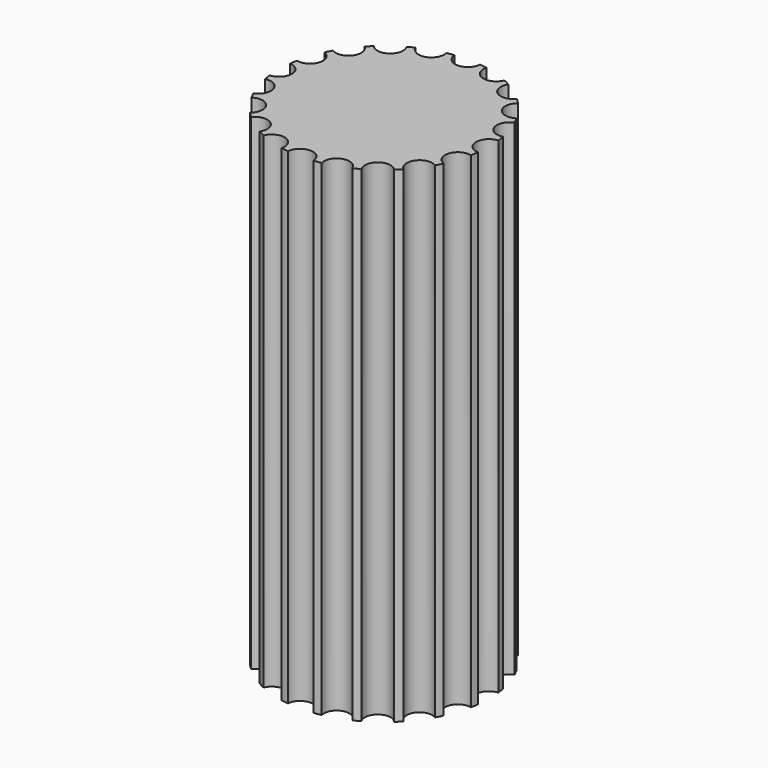
from build123d import *

# Parameters (mm, degrees)
F0_R     = 4.1
F0_R_2   = 3
F1_DEPTH = 19
F3_DEPTH = 25


with BuildPart() as f1:
    # F0 (on Top) → F1 (new body)
    with BuildSketch(Plane.XY):
        Circle(F0_R)
        Circle(F0_R_2, mode=Mode.SUBTRACT)
        Circle(F0_R_2)
    extrude(amount=F1_DEPTH)

    # F2 (on face) → F3 (cut)
    with BuildSketch(Plane.XY.offset(19)):
        with BuildLine():
            ThreePointArc((0.4990696282, 4.0695121951), (0.4997673529, 4.0847490014), (0.5, 4.1))
            ThreePointArc((0.5, 4.1), (-0.0152509986, 4.5997673529), (-0.4990696282, 4.0695121951))
            ThreePointArc((-0.4990696282, 4.0695121951), (0, 4.1), (0.4990696282, 4.0695121951))
        make_face()
        with BuildLine():
            ThreePointArc((0.4990696282, 4.0695121951), (0, 4.1), (-0.4990696282, 4.0695121951))
            ThreePointArc((-0.4990696282, 4.0695121951), (0, 3.6), (0.4990696282, 4.0695121951))
        make_face()
        with BuildLine():
            ThreePointArc((-1.7321918491, 3.7161150948), (-1.2669696769, 3.8993317168), (-0.7829050052, 4.0245570878))
            ThreePointArc((-0.7829050052, 4.0245570878), (-1.4214781741, 4.374859975), (-1.7321918491, 3.7161150948))
        make_face()
        with BuildLine():
            ThreePointArc((-0.7669696769, 3.8993317168), (-0.7709695076, 3.9624493218), (-0.7829050052, 4.0245570878))
            ThreePointArc((-0.7829050052, 4.0245570878), (-1.2669696769, 3.8993317168), (-1.7321918491, 3.7161150948))
            ThreePointArc((-1.7321918491, 3.7161150948), (-1.1737256049, 3.4081031111), (-0.7669696769, 3.8993317168))
        make_face()
        with BuildLine():
            ThreePointArc((1.7321918491, 3.7161150948), (1.2669696769, 3.8993317168), (0.7829050052, 4.0245570878))
            ThreePointArc((0.7829050052, 4.0245570878), (1.1124611797, 3.4238034587), (1.7321918491, 3.7161150948))
        make_face()
        with BuildLine():
            ThreePointArc((-2.7957550629, 2.9989587574), (-2.4099195344, 3.3169696769), (-1.9882434418, 3.585650292))
            ThreePointArc((-1.9882434418, 3.585650292), (-2.7038121605, 3.7214781741), (-2.7957550629, 2.9989587574))
        make_face()
        with BuildLine():
            ThreePointArc((-1.9099195344, 3.3169696769), (-1.929899719, 3.4569017206), (-1.9882434418, 3.585650292))
            ThreePointArc((-1.9882434418, 3.585650292), (-2.4099195344, 3.3169696769), (-2.7957550629, 2.9989587574))
            ThreePointArc((-2.7957550629, 2.9989587574), (-2.2409783675, 2.8463754971), (-1.9099195344, 3.3169696769))
        make_face()
        with BuildLine():
            ThreePointArc((2.7957550629, 2.9989587574), (2.4099195344, 3.3169696769), (1.9882434418, 3.585650292))
            ThreePointArc((1.9882434418, 3.585650292), (2.1160269083, 2.9124611797), (2.7957550629, 2.9989587574))
        make_face()
        with BuildLine():
            ThreePointArc((-3.585650292, 1.9882434418), (-3.3169696769, 2.4099195344), (-2.9989587574, 2.7957550629))
            ThreePointArc((-2.9989587574, 2.7957550629), (-3.7214781741, 2.7038121605), (-3.585650292, 1.9882434418))
        make_face()
        with BuildLine():
            ThreePointArc((-2.8169696769, 2.4099195344), (-2.8647498964, 2.6232204254), (-2.9989587574, 2.7957550629))
            ThreePointArc((-2.9989587574, 2.7957550629), (-3.3169696769, 2.4099195344), (-3.585650292, 1.9882434418))
            ThreePointArc((-3.585650292, 1.9882434418), (-3.0764913073, 1.9715473709), (-2.8169696769, 2.4099195344))
        make_face()
        with BuildLine():
            ThreePointArc((3.585650292, 1.9882434418), (3.3169696769, 2.4099195344), (2.9989587574, 2.7957550629))
            ThreePointArc((2.9989587574, 2.7957550629), (2.9124611797, 2.1160269083), (3.585650292, 1.9882434418))
        make_face()
        with BuildLine():
            ThreePointArc((-4.0245570878, 0.7829050052), (-3.8993317168, 1.2669696769), (-3.7161150948, 1.7321918491))
            ThreePointArc((-3.7161150948, 1.7321918491), (-4.374859975, 1.4214781741), (-4.0245570878, 0.7829050052))
        make_face()
        with BuildLine():
            ThreePointArc((-3.3993317168, 1.2669696769), (-3.486047123, 1.5483872395), (-3.7161150948, 1.7321918491))
            ThreePointArc((-3.7161150948, 1.7321918491), (-3.8993317168, 1.2669696769), (-4.0245570878, 0.7829050052))
            ThreePointArc((-4.0245570878, 0.7829050052), (-3.5932375201, 0.8716137073), (-3.3993317168, 1.2669696769))
        make_face()
        with BuildLine():
            ThreePointArc((4.0245570878, 0.7829050052), (3.8993317168, 1.2669696769), (3.7161150948, 1.7321918491))
            ThreePointArc((3.7161150948, 1.7321918491), (3.4238034587, 1.1124611797), (4.0245570878, 0.7829050052))
        make_face()
        with BuildLine():
            ThreePointArc((-4.0695121951, -0.4990696282), (-4.1, 0), (-4.0695121951, 0.4990696282))
            ThreePointArc((-4.0695121951, 0.4990696282), (-4.6, 0), (-4.0695121951, -0.4990696282))
        make_face()
        with BuildLine():
            ThreePointArc((-3.6, 0), (-3.7358270312, 0.3426047997), (-4.0695121951, 0.4990696282))
            ThreePointArc((-4.0695121951, 0.4990696282), (-4.1, 0), (-4.0695121951, -0.4990696282))
            ThreePointArc((-4.0695121951, -0.4990696282), (-3.7358270312, -0.3426047997), (-3.6, 0))
        make_face()
        with BuildLine():
            ThreePointArc((4.1, 0), (4.0923709509, 0.25), (4.0695121951, 0.4990696282))
            ThreePointArc((4.0695121951, 0.4990696282), (3.6, 0), (4.0695121951, -0.4990696282))
            ThreePointArc((4.0695121951, -0.4990696282), (4.0923709509, -0.25), (4.1, 0))
        make_face()
        with BuildLine():
            ThreePointArc((4.6, 0), (4.4426047997, 0.3641729688), (4.0695121951, 0.4990696282))
            ThreePointArc((4.0695121951, 0.4990696282), (4.0923709509, 0.25), (4.1, 0))
            ThreePointArc((4.1, 0), (4.0923709509, -0.25), (4.0695121951, -0.4990696282))
            ThreePointArc((4.0695121951, -0.4990696282), (4.4426047997, -0.3641729688), (4.6, 0))
        make_face()
        with BuildLine():
            ThreePointArc((-3.7161150948, -1.7321918491), (-3.8993317168, -1.2669696769), (-4.0245570878, -0.7829050052))
            ThreePointArc((-4.0245570878, -0.7829050052), (-4.374859975, -1.4214781741), (-3.7161150948, -1.7321918491))
        make_face()
        with BuildLine():
            ThreePointArc((-3.3993317168, -1.2669696769), (-3.5932375201, -0.8716137073), (-4.0245570878, -0.7829050052))
            ThreePointArc((-4.0245570878, -0.7829050052), (-3.8993317168, -1.2669696769), (-3.7161150948, -1.7321918491))
            ThreePointArc((-3.7161150948, -1.7321918491), (-3.486047123, -1.5483872395), (-3.3993317168, -1.2669696769))
        make_face()
        with BuildLine():
            ThreePointArc((3.7161150948, -1.7321918491), (3.8993317168, -1.2669696769), (4.0245570878, -0.7829050052))
            ThreePointArc((4.0245570878, -0.7829050052), (3.4238034587, -1.1124611797), (3.7161150948, -1.7321918491))
        make_face()
        with BuildLine():
            ThreePointArc((-2.8169696769, -2.4099195344), (-3.0764913073, -1.9715473709), (-3.585650292, -1.9882434418))
            ThreePointArc((-3.585650292, -1.9882434418), (-3.3169696769, -2.4099195344), (-2.9989587574, -2.7957550629))
            ThreePointArc((-2.9989587574, -2.7957550629), (-2.8647498964, -2.6232204254), (-2.8169696769, -2.4099195344))
        make_face()
        with BuildLine():
            ThreePointArc((2.9989587574, -2.7957550629), (3.3169696769, -2.4099195344), (3.585650292, -1.9882434418))
            ThreePointArc((3.585650292, -1.9882434418), (2.9124611797, -2.1160269083), (2.9989587574, -2.7957550629))
        make_face()
        with BuildLine():
            ThreePointArc((-1.9099195344, -3.3169696769), (-2.2409783675, -2.8463754971), (-2.7957550629, -2.9989587574))
            ThreePointArc((-2.7957550629, -2.9989587574), (-2.4099195344, -3.3169696769), (-1.9882434418, -3.585650292))
            ThreePointArc((-1.9882434418, -3.585650292), (-1.929899719, -3.4569017206), (-1.9099195344, -3.3169696769))
        make_face()
        with BuildLine():
            ThreePointArc((1.9882434418, -3.585650292), (2.4099195344, -3.3169696769), (2.7957550629, -2.9989587574))
            ThreePointArc((2.7957550629, -2.9989587574), (2.1160269083, -2.9124611797), (1.9882434418, -3.585650292))
        make_face()
        with BuildLine():
            ThreePointArc((-0.7669696769, -3.8993317168), (-1.1737256049, -3.4081031111), (-1.7321918491, -3.7161150948))
            ThreePointArc((-1.7321918491, -3.7161150948), (-1.2669696769, -3.8993317168), (-0.7829050052, -4.0245570878))
            ThreePointArc((-0.7829050052, -4.0245570878), (-0.7709695076, -3.9624493218), (-0.7669696769, -3.8993317168))
        make_face()
        with BuildLine():
            ThreePointArc((0.7829050052, -4.0245570878), (1.2669696769, -3.8993317168), (1.7321918491, -3.7161150948))
            ThreePointArc((1.7321918491, -3.7161150948), (1.1124611797, -3.4238034587), (0.7829050052, -4.0245570878))
        make_face()
        with BuildLine():
            ThreePointArc((0.4990696282, -4.0695121951), (0, -3.6), (-0.4990696282, -4.0695121951))
            ThreePointArc((-0.4990696282, -4.0695121951), (0, -4.1), (0.4990696282, -4.0695121951))
        make_face()
    extrude(amount=-F3_DEPTH, mode=Mode.SUBTRACT)


solid = f1.part
